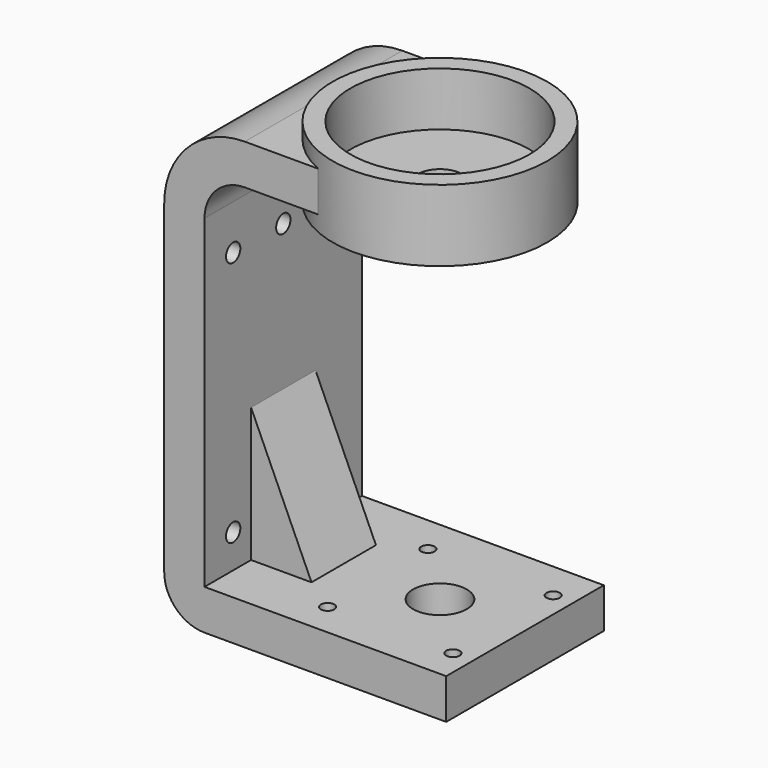
from build123d import *

# Parameters (mm, degrees)
F0_W      = 2
F0_H      = 9
F0_W_2    = 24
F1_DEPTH  = 22
F3_R      = 20
F4_DEPTH  = 12
F5_R      = 5
F5_R_2    = 4.05
F6_DEPTH  = 50
F7_R      = 2
F8_DEPTH  = 9.001
F9_R      = 11
F10_DEPTH = 2
F11_R     = 1.5
F12_DEPTH = 20
F13_R     = 6
F14_DEPTH = 25
F15_DEPTH = 9


with BuildPart() as f1:
    # F0 (on Front) → F1 (new body, symmetric)
    with BuildSketch(Plane.XZ):
        with BuildLine():
            Line((-16, 51.5), (-16, 60.5))
            ThreePointArc((-16, 60.5), (-28.7279220614, 55.2279220614), (-34, 42.5))
            Line((-34, 42.5), (-34, -30))
            ThreePointArc((-34, -30), (-31.3639610307, -36.3639610307), (-25, -39))
            Line((-25, -39), (-25, -30))
            Line((-25, -30), (-25, 0))
            Line((-25, 0), (-25, 42.5))
            ThreePointArc((-25, 42.5), (-22.3639610307, 48.8639610307), (-16, 51.5))
        make_face()
        with Locations((-15, 56)):
            Rectangle(F0_W, F0_H)
        with Locations((-2, 56)):
            Rectangle(F0_W_2, F0_H)
        Polygon((-25, -30), (-25, -39), (29, -39), (29, -30), (-11.5, -30), align=None)
    extrude(amount=F1_DEPTH, both=True)

    # F0 (on Front) → F2 (revolve)
    with BuildSketch(Plane.XZ):
        Polygon((34, 64), (10, 64), (10, 60.5), (10, 51.5), (10, 48), (34, 48), align=None)
    revolve(axis=Axis((10, 0, 55.4929765165), (0, 0, -1)))

    # F3 (on face) → F4 (cut)
    with BuildSketch(Plane.XY.offset(64)):
        with Locations((10, 0)):
            Circle(F3_R)
    extrude(amount=-F4_DEPTH, mode=Mode.SUBTRACT)

    # F5 (on face) → F6 (cut)
    with BuildSketch(Plane.XY.offset(52)):
        with Locations((10, 0)):
            Circle(F5_R)
        with Locations((20, 0)):
            Circle(F5_R_2)
    extrude(amount=-F6_DEPTH, mode=Mode.SUBTRACT)

    # F7 (on face) → F8 (cut, through all)
    with BuildSketch(Plane.YZ.offset(-25)):
        with Locations((14, -22.5)):
            Circle(F7_R)
        with Locations((14, 32.5)):
            Circle(F7_R)
        with Locations((0, 32.5)):
            Circle(F7_R)
        with Locations((-14, -22.5)):
            Circle(F7_R)
        with Locations((-14, 32.5)):
            Circle(F7_R)
    extrude(amount=-F8_DEPTH, mode=Mode.SUBTRACT)

    # F9 (on face) → F10 (cut)
    with BuildSketch(Plane(origin=(0, 0, -39), x_dir=(1, 0, 0), z_dir=(0, 0, -1))):
        with Locations((10, 0)):
            Circle(F9_R)
    extrude(amount=-F10_DEPTH, mode=Mode.SUBTRACT)

    # F11 (on face) → F12 (cut)
    with BuildSketch(Plane(origin=(0, 0, -39), x_dir=(1, 0, 0), z_dir=(0, 0, -1))):
        with Locations((-3.5, -13.5)):
            Circle(F11_R)
        with Locations((-3.5, 14.5)):
            Circle(F11_R)
        with Locations((24.5, -13.5)):
            Circle(F11_R)
        with Locations((24.5, 14.5)):
            Circle(F11_R)
        with Locations((52.5, -13.5)):
            Circle(F11_R)
        with Locations((52.5, 14.5)):
            Circle(F11_R)
    extrude(amount=-F12_DEPTH, mode=Mode.SUBTRACT)

    # F13 (on face) → F14 (cut)
    with BuildSketch(Plane(origin=(0, 0, -39), x_dir=(1, 0, 0), z_dir=(0, 0, -1))):
        with Locations((10, 0)):
            Circle(F13_R)
    extrude(amount=-F14_DEPTH, mode=Mode.SUBTRACT)

    # F0 (on Front) → F15 (join, symmetric)
    with BuildSketch(Plane.XZ):
        Polygon((-11.5, -30), (-25, 0), (-25, -30), align=None)
    extrude(amount=F15_DEPTH, both=True)


solid = f1.part
